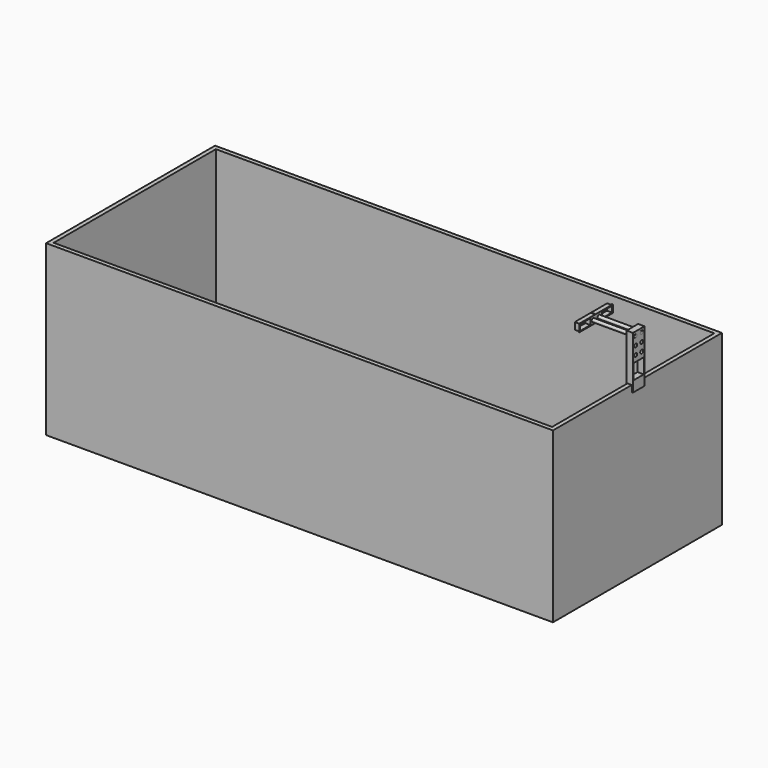
from build123d import *

# Parameters (mm, degrees)
F0_W          = 1.5
F0_H          = 1
F0_H_2        = 16
F0_R          = 4.25
F0_W_2        = 30
F0_H_3        = 14
F1_DEPTH      = 2
F2_DEPTH      = 10
F2_DEPTH_BACK = 2
F5_W          = 1200
F5_H          = 500
F5_W_2        = 1180
F5_H_2        = 480
F6_DEPTH      = 400
F7_W          = 10
F7_H          = 2
F7_W_2        = 1
F7_H_2        = 30
F8_DEPTH      = 10
F9_DEPTH      = 15
F10_R         = 4.25
F11_DEPTH     = 15
F12_W         = 110
F12_H         = 4


# Not quite as in the source:
# - a feature names something its author has since deleted; it is built from what else it names
# - the program builds the solid bodies; features that only make, move or delete a surface that nothing else refers to are left out


with BuildPart() as f1:
    # F0 (on Right) → F1 (new body)
    with BuildSketch(Plane.YZ):
        Polygon((-0.75, 9), (-49.5, 9), (-49.5, -9), (-0.75, -9), (-0.75, -8), (-13, -8), (-16, -8), (-48, -8), (-48, 8), (-16, 8), (-13, 8), (-0.75, 8), align=None)
        with Locations((0, 8.5)):
            Rectangle(F0_W, F0_H)
        Polygon((49.5, 9), (0.75, 9), (0.75, 8), (13, 8), (16, 8), (48, 8), (48, -8), (16, -8), (13, -8), (0.75, -8), (0.75, -9), (49.5, -9), align=None)
        with Locations((0, -8.5)):
            Rectangle(F0_W, F0_H)
        Rectangle(F0_W, F0_H_2)
        Polygon((13, 8), (0.75, 8), (0.75, -8), (13, -8), (16, -8), (48, -8), (48, 8), (16, 8), align=None)
        with Locations((8.75, 0)):
            Circle(F0_R, mode=Mode.SUBTRACT)
        with Locations((32, 0)):
            Rectangle(F0_W_2, F0_H_3, mode=Mode.SUBTRACT)
    extrude(amount=F1_DEPTH)

    # F0 (on Right) → F2 (join, two sides)
    with BuildSketch(Plane.YZ) as f2_sk:
        Polygon((-0.75, -8), (-0.75, 8), (-13, 8), (-16, 8), (-48, 8), (-48, -8), (-16, -8), (-13, -8), align=None)
        with Locations((-32, 0)):
            Rectangle(F0_W_2, F0_H_3, mode=Mode.SUBTRACT)
        with Locations((-8.75, 0)):
            Circle(F0_R, mode=Mode.SUBTRACT)
        Polygon((13, 8), (0.75, 8), (0.75, -8), (13, -8), (16, -8), (48, -8), (48, 8), (16, 8), align=None)
        with Locations((8.75, 0)):
            Circle(F0_R, mode=Mode.SUBTRACT)
        with Locations((32, 0)):
            Rectangle(F0_W_2, F0_H_3, mode=Mode.SUBTRACT)
    extrude(amount=-F2_DEPTH)
    extrude(f2_sk.sketch, amount=F2_DEPTH_BACK)


with BuildPart() as f6:
    # F5 (on offset) → F6 (new body)
    with BuildSketch(Plane.XY.offset(-500)):
        with Locations((-500, 0)):
            Rectangle(F5_W, F5_H)
        with Locations((-500, 0)):
            Rectangle(F5_W_2, F5_H_2, mode=Mode.SUBTRACT)
    extrude(amount=F6_DEPTH)


with BuildPart() as f8:
    # F7 (on face) → F8 (new body)
    with BuildSketch(Plane.XY.offset(-100)):
        Polygon((101, 17), (101, 15), (101, -15), (101, -17), (103, -17), (103, 17), align=None)
        Polygon((90, -15), (90, 15), (90, 17), (88, 17), (88, -17), (90, -17), align=None)
        with Locations((95, 16)):
            Rectangle(F7_W, F7_H)
        with Locations((100.5, 16)):
            Rectangle(F7_W_2, F7_H)
        with Locations((100.5, -16)):
            Rectangle(F7_W_2, F7_H)
        with Locations((95, -16)):
            Rectangle(F7_W, F7_H)
        with Locations((100.5, 0)):
            Rectangle(F7_W_2, F7_H_2)
        with Locations((95, 0)):
            Rectangle(F7_W, F7_H_2)
    extrude(amount=F8_DEPTH)

    # F7 (on face) → F9 (join)
    with BuildSketch(Plane.XY.offset(-100)):
        Polygon((90, -15), (90, 15), (90, 17), (88, 17), (88, -17), (90, -17), align=None)
        Polygon((101, 17), (101, 15), (101, -15), (101, -17), (103, -17), (103, 17), align=None)
    extrude(amount=-F9_DEPTH)

    # F10 (on face) → F11 (join)
    with BuildSketch(Plane.YZ.offset(103)):
        Polygon((-15, -90), (-17, -90), (-17, -100), (17, -100), (17, -90), (15, -90), align=None)
        Polygon((-17, 9.5), (-17, -90), (-15, -90), (-15, -54.25), (15, -54.25), (15, -90), (17, -90), (17, 9.5), align=None)
        with Locations((-8.75, -40)):
            Circle(F10_R, mode=Mode.SUBTRACT)
        with Locations((-8.75, -20)):
            Circle(F10_R, mode=Mode.SUBTRACT)
        with Locations((-8.75, 0)):
            Circle(F10_R, mode=Mode.SUBTRACT)
        with Locations((8.75, -40)):
            Circle(F10_R, mode=Mode.SUBTRACT)
        with Locations((8.75, -20)):
            Circle(F10_R, mode=Mode.SUBTRACT)
        with Locations((8.75, 0)):
            Circle(F10_R, mode=Mode.SUBTRACT)
    extrude(amount=-F11_DEPTH)


with BuildPart() as f13:
    # F12 (on Top) → F13 (revolve)
    with BuildSketch(Plane.XY):
        with Locations((48, -6.5)):
            Rectangle(F12_W, F12_H)
    revolve(axis=Axis((48, -8.5, 0), (1, 0, 0)))


with BuildPart() as f14:
    # F12 (on Top) → F14 (revolve)
    with BuildSketch(Plane.XY):
        with Locations((48, 6.5)):
            Rectangle(F12_W, F12_H)
    revolve(axis=Axis((48, 8.5, 0), (1, 0, 0)))


solid = Compound([f1.part, f6.part, f8.part, f13.part, f14.part])
